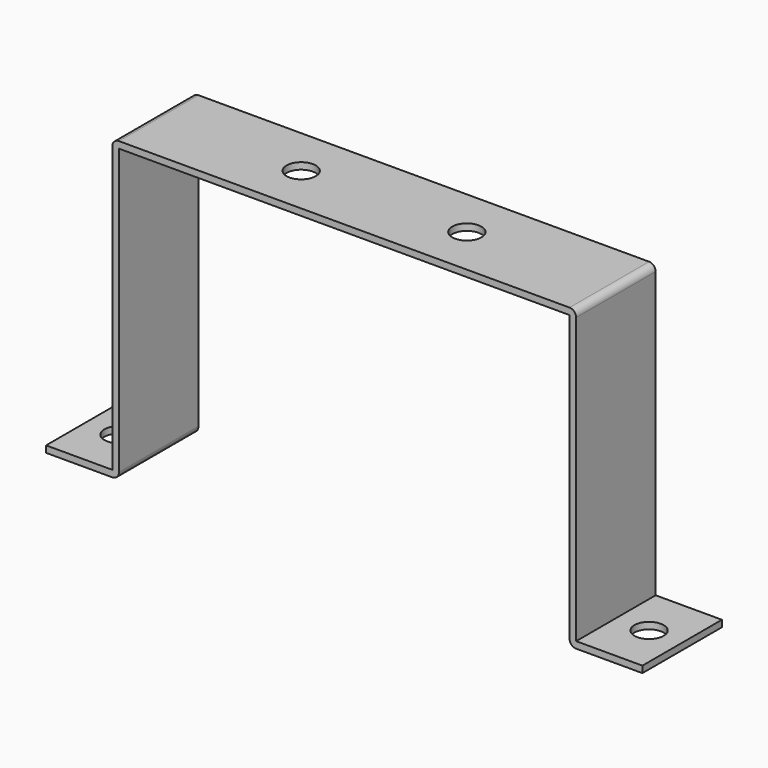
from build123d import *

# Parameters (mm, degrees)
F1_DEPTH = 30
F2_R     = 4.4
F3_R     = 4.4
F4_DEPTH = 25
F5_R     = 2
F6_R     = 2


# Not quite as in the source:
# - a feature names something its author has since deleted; it is built from what else it names


with BuildPart() as f1:
    # F0 (on Front) → F1 (new body)
    with BuildSketch(Plane.XZ):
        Polygon((90, -1), (90, 1), (70, 1), (70, 89), (-70, 89), (-70, 1), (-90, 1), (-90, -1), (-68, -1), (-68, 87), (68, 87), (68, -1), align=None)
    extrude(amount=F1_DEPTH)

    # F2 (on face) + F3 (on face) → F4 (cut)
    with BuildSketch(Plane.XY.offset(1)):
        with Locations((-80, -15)):
            Circle(F2_R)
        with Locations((80, -15)):
            Circle(F2_R)
    with BuildSketch(Plane.XY.offset(89)):
        with Locations((-25, -15)):
            Circle(F3_R)
        with Locations((25, -15)):
            Circle(F3_R)
    extrude(amount=-F4_DEPTH, mode=Mode.SUBTRACT)

    # F5
    f5_edges = [f1.edges().sort_by_distance(p)[0] for p in [
        (-70, -15, 89),
        (70, -15, 89),
    ]]
    fillet(f5_edges, radius=F5_R)

    # F6
    f6_edges = [f1.edges().sort_by_distance(p)[0] for p in [
        (68, -15, -1),
        (-68, -15, -1),
    ]]
    fillet(f6_edges, radius=F6_R)


solid = f1.part
